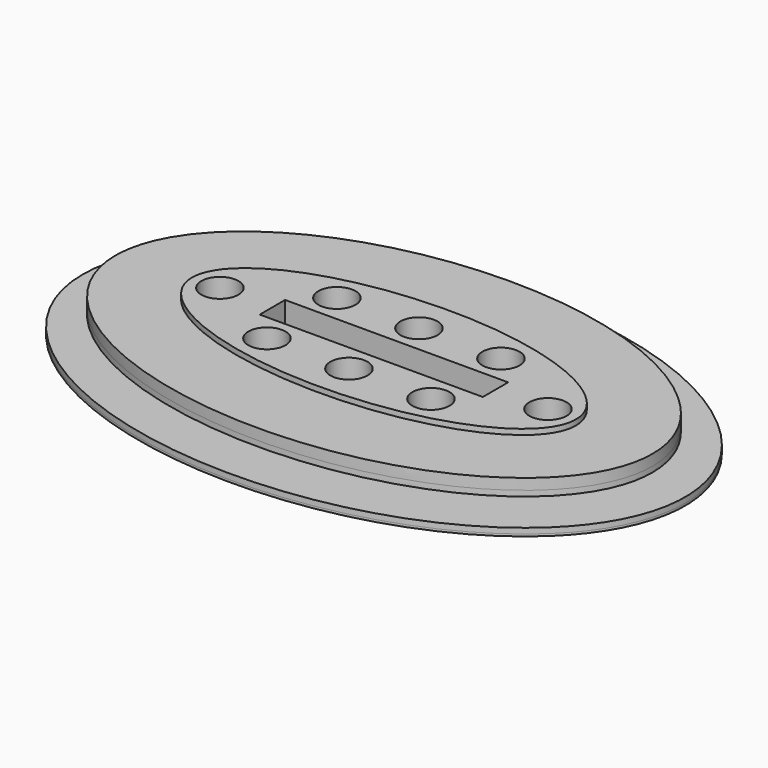
from build123d import *

# Parameters (mm, degrees)
F1_DEPTH  = 2
F3_DEPTH  = 0.5
F5_DEPTH  = 1.5
F7_R      = 1.7
F8_DEPTH  = 2.3
F10_DEPTH = 0.5
F12_DEPTH = 0.2
F6_W      = 20.4
F6_H      = 2.9
F13_DEPTH = 3.2
F14_W     = 19.45
F14_H     = 1.7
F15_DEPTH = 1
F17_DEPTH = 1
F19_DEPTH = 0.2


# Not quite as in the source:
# - a feature names something its author has since deleted; it is built from what else it names


with BuildPart() as f1:
    # F0 (on Top) → F1 (new body)
    with BuildSketch(Plane.XY):
        with BuildLine():
            add(Edge.make_bspline(
                [(-17.556335, 39.4589360392), (-17.556335, 26.4777608324), (8.7781675, 32.9683484358), (35.11267, 39.4589360392), (8.7781675, 45.9495236425), (-17.556335, 52.4401112459), (-17.556335, 39.4589360392)],
                knots=[0, 0, 0, 2.0943951024, 2.0943951024, 4.1887902048, 4.1887902048, 6.2831853072, 6.2831853072, 6.2831853072], degree=2, weights=[1, 0.5, 1, 0.5, 1, 0.5, 1]))
        make_face()
    extrude(amount=-F1_DEPTH)

    # F2 (on face) → F3 (join)
    with BuildSketch(Plane.XY):
        with BuildLine():
            add(Edge.make_bspline(
                [(-24.556335, 39.4589360392), (-24.556335, 14.3534051795), (12.2781675, 26.9061706093), (49.11267, 39.4589360392), (12.2781675, 52.011701469), (-24.556335, 64.5644668989), (-24.556335, 39.4589360392)],
                knots=[0, 0, 0, 2.0943951024, 2.0943951024, 4.1887902048, 4.1887902048, 6.2831853072, 6.2831853072, 6.2831853072], degree=2, weights=[1, 0.5, 1, 0.5, 1, 0.5, 1]))
        make_face()
    extrude(amount=-F3_DEPTH)

    # F4 (on face) → F5 (join)
    with BuildSketch(Plane.XY):
        with BuildLine():
            add(Edge.make_bspline(
                [(-17.556335, 39.4589360392), (-17.556335, 26.4777608324), (8.7781675, 32.9683484358), (35.11267, 39.4589360392), (8.7781675, 45.9495236425), (-17.556335, 52.4401112459), (-17.556335, 39.4589360392)],
                knots=[0, 0, 0, 2.0943951024, 2.0943951024, 4.1887902048, 4.1887902048, 6.2831853072, 6.2831853072, 6.2831853072], degree=2, weights=[1, 0.5, 1, 0.5, 1, 0.5, 1]))
        make_face()
    extrude(amount=F5_DEPTH)

    # F7 (on face) → F8 (cut)
    with BuildSketch(Plane.XY.offset(1.5)):
        with Locations((-15, 39.4589360392)):
            Circle(F7_R)
        with Locations((0, 43.4589360392)):
            Circle(F7_R)
        with Locations((15, 39.4589360392)):
            Circle(F7_R)
        with Locations((0, 35.4589360392)):
            Circle(F7_R)
        with Locations((-7.5, 35.4589360392)):
            Circle(F7_R)
        with Locations((-7.5, 43.4589360392)):
            Circle(F7_R)
        with Locations((7.5, 43.4589360392)):
            Circle(F7_R)
        with Locations((7.5, 35.4589360392)):
            Circle(F7_R)
    extrude(amount=-F8_DEPTH, mode=Mode.SUBTRACT)

    # F9 (on face) → F10 (join)
    with BuildSketch(Plane(origin=(0, 0, -2), x_dir=(1, 0, 0), z_dir=(0, 0, -1))):
        with BuildLine():
            add(Edge.make_bspline(
                [(-27.556335, -39.4589360392), (-27.556335, -69.7606193216), (13.7781675, -54.6097776804), (55.11267, -39.4589360392), (13.7781675, -24.308094398), (-27.556335, -9.1572527567), (-27.556335, -39.4589360392)],
                knots=[0, 0, 0, 2.0943951024, 2.0943951024, 4.1887902048, 4.1887902048, 6.2831853072, 6.2831853072, 6.2831853072], degree=2, weights=[1, 0.5, 1, 0.5, 1, 0.5, 1]))
        make_face()
    extrude(amount=-F10_DEPTH)

    # F11 (on face) → F12 (join)
    with BuildSketch(Plane(origin=(0, 0, -2), x_dir=(1, 0, 0), z_dir=(0, 0, -1))):
        with BuildLine():
            add(Edge.make_bspline(
                [(-17.556335, -39.4589360392), (-17.556335, -52.4401112459), (8.7781675, -45.9495236425), (35.11267, -39.4589360392), (8.7781675, -32.9683484358), (-17.556335, -26.4777608324), (-17.556335, -39.4589360392)],
                knots=[0, 0, 0, 2.0943951024, 2.0943951024, 4.1887902048, 4.1887902048, 6.2831853072, 6.2831853072, 6.2831853072], degree=2, weights=[1, 0.5, 1, 0.5, 1, 0.5, 1]))
        make_face()
    extrude(amount=F12_DEPTH)

    # F6 (on face) → F13 (cut)
    with BuildSketch(Plane.XY.offset(1.5)):
        with Locations((0, 39.4589360392)):
            Rectangle(F6_W, F6_H)
    extrude(amount=-F13_DEPTH, mode=Mode.SUBTRACT)

    # F14 (on face) → F15 (cut)
    with BuildSketch(Plane.XY.offset(-1.7)):
        with Locations((0, 39.4839360392)):
            Rectangle(F14_W, F14_H)
    extrude(amount=-F15_DEPTH, mode=Mode.SUBTRACT)

    # F16 (on face) → F17 (join)
    with BuildSketch(Plane.XY):
        with BuildLine():
            add(Edge.make_bspline(
                [(-24.556335, 39.4589360392), (-24.556335, 14.3534051795), (12.2781675, 26.9061706093), (49.11267, 39.4589360392), (12.2781675, 52.011701469), (-24.556335, 64.5644668989), (-24.556335, 39.4589360392)],
                knots=[0, 0, 0, 2.0943951024, 2.0943951024, 4.1887902048, 4.1887902048, 6.2831853072, 6.2831853072, 6.2831853072], degree=2, weights=[1, 0.5, 1, 0.5, 1, 0.5, 1]))
        make_face()
        with BuildLine():
            add(Edge.make_bspline(
                [(-17.556335, 39.4589360392), (-17.556335, 26.4777608324), (8.7781675, 32.9683484358), (35.11267, 39.4589360392), (8.7781675, 45.9495236425), (-17.556335, 52.4401112459), (-17.556335, 39.4589360392)],
                knots=[0, 0, 0, 2.0943951024, 2.0943951024, 4.1887902048, 4.1887902048, 6.2831853072, 6.2831853072, 6.2831853072], degree=2, weights=[1, 0.5, 1, 0.5, 1, 0.5, 1]))
        make_face(mode=Mode.SUBTRACT)
    extrude(amount=F17_DEPTH)

    # F18 (on face) → F19 (join)
    with BuildSketch(Plane(origin=(0, 0, -2), x_dir=(1, 0, 0), z_dir=(0, 0, -1))):
        with BuildLine():
            add(Edge.make_bspline(
                [(-27.556335, -39.4589360392), (-27.556335, -69.7606193216), (13.7781675, -54.6097776804), (55.11267, -39.4589360392), (13.7781675, -24.308094398), (-27.556335, -9.1572527567), (-27.556335, -39.4589360392)],
                knots=[0, 0, 0, 2.0943951024, 2.0943951024, 4.1887902048, 4.1887902048, 6.2831853072, 6.2831853072, 6.2831853072], degree=2, weights=[1, 0.5, 1, 0.5, 1, 0.5, 1]))
        make_face()
        with BuildLine():
            add(Edge.make_bspline(
                [(-17.556335, -39.4589360392), (-17.556335, -52.4401112459), (8.7781675, -45.9495236425), (35.11267, -39.4589360392), (8.7781675, -32.9683484358), (-17.556335, -26.4777608324), (-17.556335, -39.4589360392)],
                knots=[0, 0, 0, 2.0943951024, 2.0943951024, 4.1887902048, 4.1887902048, 6.2831853072, 6.2831853072, 6.2831853072], degree=2, weights=[1, 0.5, 1, 0.5, 1, 0.5, 1]))
        make_face(mode=Mode.SUBTRACT)
    extrude(amount=F19_DEPTH)


solid = f1.part
